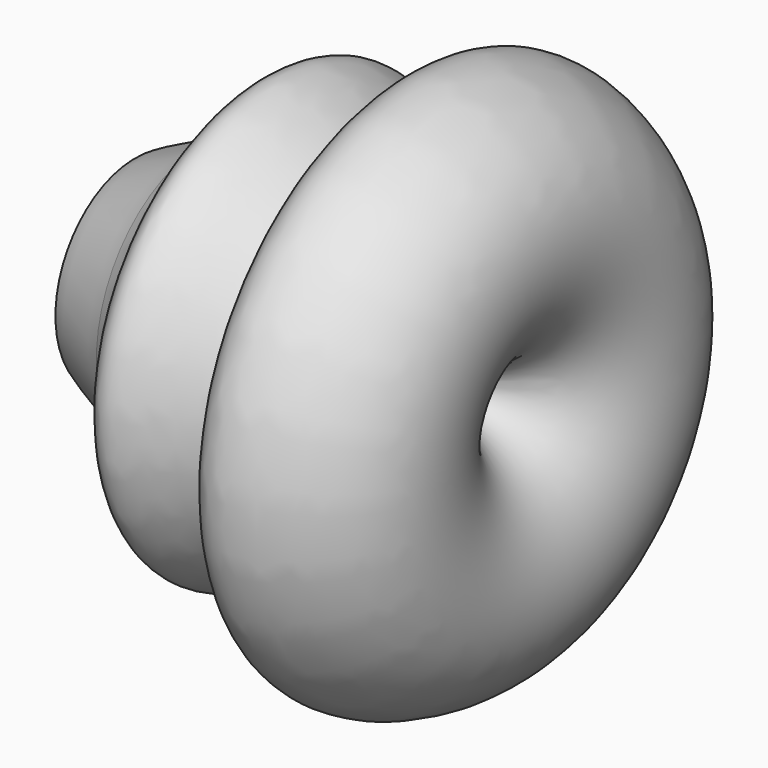
from build123d import *


with BuildPart() as f1:
    # F0 (on Top) → F1 (revolve)
    with BuildSketch(Plane.XY):
        with BuildLine():
            add(Edge.make_bspline(
                [(-41.0288795829, 40.0111079216), (-35.0517399376, 43.7348528862), (-31.3081519856, 50.7803672753), (-24.5920273822, 65.2547737041), (-2.5115567987, 45.9401566124), (4.3152030161, 46.8650144905), (0.9176389649, 57.1238671779), (5.6913339977, 77.9902599803), (44.0273149346, 61.8230874277), (41.1015782973, 21.6662005598), (15.9059542904, 9.813878531), (4.25732443, 8.9691039175)],
                knots=[0, 0, 0, 0, 0.0648058033, 0.1172723616, 0.1993880152, 0.2326801218, 0.2822612272, 0.3465359592, 0.4361506248, 0.5315351097, 0.6191355146, 0.6191355146, 0.6191355146, 0.6191355146], degree=3))
            add(Edge.make_bspline(
                [(-1.6919113884, 8.9691039175), (-1.7527229599, 8.9737080062), (-10.449175789, 9.6534153588), (-25.553078222, 16.7093559916), (-0.6185701006, 18.6758424913), (-2.8518552938, 37.9236040107), (-76.8762743567, 25.7961258741), (-47.5074669732, 35.9749621054), (-41.0288795829, 40.0111079216)],
                knots=[0.6342141624, 0.6342141624, 0.6342141624, 0.6342141624, 0.6346840769, 0.7014595804, 0.7635522232, 0.813650341, 0.9297573614, 1, 1, 1, 1], degree=3))
            Line((-1.6919113884, 8.9691039175), (4.25732443, 8.9691039175))
        make_face()
    revolve(axis=Axis((18.5107029974, 8.9691039175, 0), (1, 0, 0)))


with BuildPart() as f1_1:
    # F2: moved
    add(f1.part.moved(Location((0, 0, 50))))


solid = f1_1.part
